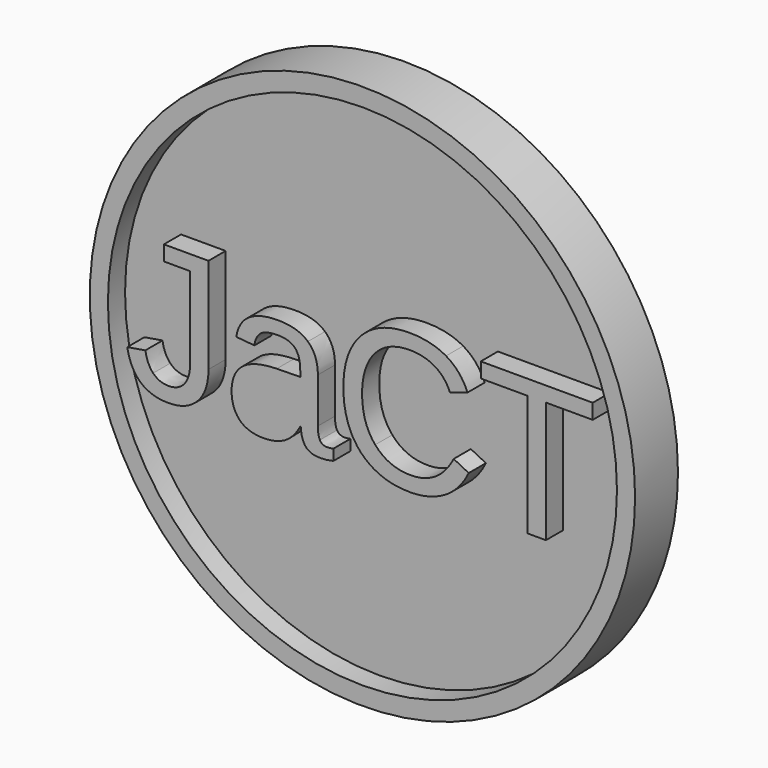
from build123d import *

# Parameters (mm, degrees)
F0_R      = 25.4414928825
F1_DEPTH  = 5
F2_R      = 23.75
F3_DEPTH  = 2
F4_W      = 4.6242554672
F4_H      = 13.1795220077
F5_DEPTH  = 5
F6_R      = 1
F8_D      = 3
F9_W      = 33.4208746554
F9_H      = 3.9936437383
F10_DEPTH = 5
F11_R     = 1.5
F12_R     = 1


with BuildPart() as f1:
    # F0 (on Front) → F1 (new body)
    with BuildSketch(Plane.XZ):
        Circle(F0_R)
    extrude(amount=F1_DEPTH)

    # F2 (on face) → F3 (cut)
    with BuildSketch(Plane.XZ.offset(5)):
        Circle(F2_R)
        with BuildLine():
            add(Edge.make_bspline(
                [(-7.2510674036, -5.9716344181), (-8.0767025075, -6.4364150185), (-9.2574184429, -6.4364150185)],
                knots=[0, 0, 0, 1, 1, 1], degree=2))
            add(Edge.make_bspline(
                [(-9.2574184429, -6.4364150185), (-10.729704817, -6.4364150185), (-11.4687348401, -5.6598561271)],
                knots=[0, 0, 0, 1, 1, 1], degree=2))
            add(Edge.make_bspline(
                [(-11.4687348401, -5.6598561271), (-12.2077648632, -4.8832972356), (-12.2077648632, -3.5293711386)],
                knots=[0, 0, 0, 1, 1, 1], degree=2))
            add(Edge.make_bspline(
                [(-12.2077648632, -3.5293711386), (-12.2077648632, -2.0137822241), (-11.2103630156, -1.2025813003)],
                knots=[0, 0, 0, 1, 1, 1], degree=2))
            add(Edge.make_bspline(
                [(-11.2103630156, -1.2025813003), (-10.212961168, -0.3913803765), (-7.9958710988, -0.336530492)],
                knots=[0, 0, 0, 1, 1, 1], degree=2))
            Line((-7.9958710988, -0.336530492), (-5.8018757177, -0.2990016236))
            Line((-5.8018757177, -0.2990016236), (-5.8018757177, 0.2321762055))
            add(Edge.make_bspline(
                [(-5.8018757177, 0.2321762055), (-5.8018757177, 1.4215526489), (-6.3070720225, 1.9368528798)],
                knots=[0, 0, 0, 1, 1, 1], degree=2))
            add(Edge.make_bspline(
                [(-6.3070720225, 1.9368528798), (-6.8122683274, 2.4521531108), (-7.8948318378, 2.4521531108)],
                knots=[0, 0, 0, 1, 1, 1], degree=2))
            add(Edge.make_bspline(
                [(-7.8948318378, 2.4521531108), (-8.9860558563, 2.4521531108), (-9.482591653, 2.0811946812)],
                knots=[0, 0, 0, 1, 1, 1], degree=2))
            add(Edge.make_bspline(
                [(-9.482591653, 2.0811946812), (-9.9791274498, 1.7102362517), (-10.0801667108, 0.8990353279)],
                knots=[0, 0, 0, 1, 1, 1], degree=2))
            Line((-10.0801667108, 0.8990353279), (-11.774739459, 1.0520376373))
            add(Edge.make_bspline(
                [(-11.774739459, 1.0520376373), (-11.359035071, 3.6877189307), (-7.8601898055, 3.6877189307)],
                knots=[0, 0, 0, 1, 1, 1], degree=2))
            add(Edge.make_bspline(
                [(-7.8601898055, 3.6877189307), (-6.0183884198, 3.6877189307), (-5.0902706369, 2.8433193925)],
                knots=[0, 0, 0, 1, 1, 1], degree=2))
            add(Edge.make_bspline(
                [(-5.0902706369, 2.8433193925), (-4.162152854, 1.9989198544), (-4.162152854, 0.4024995311)],
                knots=[0, 0, 0, 1, 1, 1], degree=2))
            Line((-4.162152854, 0.4024995311), (-4.162152854, -3.8007337252))
            add(Edge.make_bspline(
                [(-4.162152854, -3.8007337252), (-4.162152854, -4.5224427322), (-3.9716216761, -4.8876274897)],
                knots=[0, 0, 0, 1, 1, 1], degree=2))
            add(Edge.make_bspline(
                [(-3.9716216761, -4.8876274897), (-3.7810904983, -5.2528122472), (-3.2499126692, -5.2528122472)],
                knots=[0, 0, 0, 1, 1, 1], degree=2))
            add(Edge.make_bspline(
                [(-3.2499126692, -5.2528122472), (-3.016078951, -5.2528122472), (-2.7187348401, -5.1893018546)],
                knots=[0, 0, 0, 1, 1, 1], degree=2))
            Line((-2.7187348401, -5.1893018546), (-2.7187348401, -6.1996944643))
            add(Edge.make_bspline(
                [(-2.7187348401, -6.1996944643), (-3.330744078, -6.3440362657), (-3.9716216761, -6.3440362657)],
                knots=[0, 0, 0, 1, 1, 1], degree=2))
            add(Edge.make_bspline(
                [(-3.9716216761, -6.3440362657), (-4.8723145168, -6.3440362657), (-5.2836886507, -5.8705951571)],
                knots=[0, 0, 0, 1, 1, 1], degree=2))
            add(Edge.make_bspline(
                [(-5.2836886507, -5.8705951571), (-5.6950627847, -5.3971540486), (-5.7499126692, -4.3867614389)],
                knots=[0, 0, 0, 1, 1, 1], degree=2))
            Line((-5.7499126692, -4.3867614389), (-5.8018757177, -4.3867614389))
            add(Edge.make_bspline(
                [(-5.8018757177, -4.3867614389), (-6.4254322997, -5.5068538176), (-7.2510674036, -5.9716344181)],
                knots=[0, 0, 0, 1, 1, 1], degree=2))
        make_face(mode=Mode.SUBTRACT)
        with BuildLine():
            add(Edge.make_bspline(
                [(-15.3659634775, -5.3755027784), (-16.3676955791, -6.4364150185), (-18.1084577038, -6.4364150185)],
                knots=[0, 0, 0, 1, 1, 1], degree=2))
            add(Edge.make_bspline(
                [(-18.1084577038, -6.4364150185), (-21.3388272188, -6.4364150185), (-21.9421759486, -3.0963457345)],
                knots=[0, 0, 0, 1, 1, 1], degree=2))
            Line((-21.9421759486, -3.0963457345), (-20.2562637085, -2.8163226398))
            add(Edge.make_bspline(
                [(-20.2562637085, -2.8163226398), (-20.0917140549, -3.8642441178), (-19.5244507754, -4.4502718315)],
                knots=[0, 0, 0, 1, 1, 1], degree=2))
            add(Edge.make_bspline(
                [(-19.5244507754, -4.4502718315), (-18.957187496, -5.0362995451), (-18.0997971958, -5.0362995451)],
                knots=[0, 0, 0, 1, 1, 1], degree=2))
            add(Edge.make_bspline(
                [(-18.0997971958, -5.0362995451), (-17.1615754867, -5.0362995451), (-16.6202937316, -4.3910916929)],
                knots=[0, 0, 0, 1, 1, 1], degree=2))
            add(Edge.make_bspline(
                [(-16.6202937316, -4.3910916929), (-16.0790119764, -3.7458838407), (-16.0790119764, -2.5016575128)],
                knots=[0, 0, 0, 1, 1, 1], degree=2))
            Line((-16.0790119764, -2.5016575128), (-16.0790119764, 5.0503055357))
            Line((-16.0790119764, 5.0503055357), (-18.5241620918, 5.0503055357))
            Line((-18.5241620918, 5.0503055357), (-18.5241620918, 6.4561946812))
            Line((-18.5241620918, 6.4561946812), (-14.3642313759, 6.4561946812))
            Line((-14.3642313759, 6.4561946812), (-14.3642313759, -2.4641286444))
            add(Edge.make_bspline(
                [(-14.3642313759, -2.4641286444), (-14.3642313759, -4.3145905382), (-15.3659634775, -5.3755027784)],
                knots=[0, 0, 0, 1, 1, 1], degree=2))
        make_face(mode=Mode.SUBTRACT)
        with BuildLine():
            add(Edge.make_bspline(
                [(6.7500873308, 4.6519221639), (5.7714499174, 5.2379498775), (4.4261843285, 5.2379498775)],
                knots=[0, 0, 0, 1, 1, 1], degree=2))
            add(Edge.make_bspline(
                [(4.4261843285, 5.2379498775), (2.3159071922, 5.2379498775), (1.142408347, 3.8811369445)],
                knots=[0, 0, 0, 1, 1, 1], degree=2))
            add(Edge.make_bspline(
                [(1.142408347, 3.8811369445), (-0.0310904983, 2.5243240115), (-0.0310904983, 0.1600053048)],
                knots=[0, 0, 0, 1, 1, 1], degree=2))
            add(Edge.make_bspline(
                [(-0.0310904983, 0.1600053048), (-0.0310904983, -2.1754450416), (1.1914845594, -3.5972117853)],
                knots=[0, 0, 0, 1, 1, 1], degree=2))
            add(Edge.make_bspline(
                [(1.1914845594, -3.5972117853), (2.4140596172, -5.0189785289), (4.4983552292, -5.0189785289)],
                knots=[0, 0, 0, 1, 1, 1], degree=2))
            add(Edge.make_bspline(
                [(4.4983552292, -5.0189785289), (7.1686785548, -5.0189785289), (8.5139441437, -2.3746367275)],
                knots=[0, 0, 0, 1, 1, 1], degree=2))
            Line((8.5139441437, -2.3746367275), (9.9198332892, -3.0790247183))
            add(Edge.make_bspline(
                [(9.9198332892, -3.0790247183), (9.1346138897, -4.7216344181), (7.7142905641, -5.5790247183)],
                knots=[0, 0, 0, 1, 1, 1], degree=2))
            add(Edge.make_bspline(
                [(7.7142905641, -5.5790247183), (6.2939672384, -6.4364150185), (4.4175238204, -6.4364150185)],
                knots=[0, 0, 0, 1, 1, 1], degree=2))
            add(Edge.make_bspline(
                [(4.4175238204, -6.4364150185), (2.494891026, -6.4364150185), (1.0918887165, -5.6367614389)],
                knots=[0, 0, 0, 1, 1, 1], degree=2))
            add(Edge.make_bspline(
                [(1.0918887165, -5.6367614389), (-0.311113593, -4.8371078592), (-1.045813362, -3.3532741409)],
                knots=[0, 0, 0, 1, 1, 1], degree=2))
            add(Edge.make_bspline(
                [(-1.045813362, -3.3532741409), (-1.7805131311, -1.8694404227), (-1.7805131311, 0.1600053048)],
                knots=[0, 0, 0, 1, 1, 1], degree=2))
            add(Edge.make_bspline(
                [(-1.7805131311, 0.1600053048), (-1.7805131311, 3.199843642), (-0.1379034313, 4.9232847505)],
                knots=[0, 0, 0, 1, 1, 1], degree=2))
            add(Edge.make_bspline(
                [(-0.1379034313, 4.9232847505), (1.5047062684, 6.6467258591), (4.4088633123, 6.6467258591)],
                knots=[0, 0, 0, 1, 1, 1], degree=2))
            add(Edge.make_bspline(
                [(4.4088633123, 6.6467258591), (6.4383090398, 6.6467258591), (7.8008956449, 5.8528459514)],
                knots=[0, 0, 0, 1, 1, 1], degree=2))
            add(Edge.make_bspline(
                [(7.8008956449, 5.8528459514), (9.16348225, 5.0589660438), (9.8043598481, 3.4971877528)],
                knots=[0, 0, 0, 1, 1, 1], degree=2))
            Line((9.8043598481, 3.4971877528), (8.1704106564, 2.9573494156))
            add(Edge.make_bspline(
                [(8.1704106564, 2.9573494156), (7.7287247442, 4.0658944503), (6.7500873308, 4.6519221639)],
                knots=[0, 0, 0, 1, 1, 1], degree=2))
        make_face(mode=Mode.SUBTRACT)
        Polygon((21.4873852523, 5.0503055357), (17.1196023424, 5.0503055357), (17.1196023424, -6.2545443488), (15.4048217419, -6.2545443488), (15.4048217419, 5.0503055357), (11.039925668, 5.0503055357), (11.039925668, 6.4561946812), (21.4873852523, 6.4561946812), align=None, mode=Mode.SUBTRACT)
    extrude(amount=-F3_DEPTH, mode=Mode.SUBTRACT)

    # F4 (on face) → F5 (join)
    with BuildSketch(Plane(origin=(0, 0, 0), x_dir=(-1, 0, 0), z_dir=(0, 1, 0))):
        with Locations((8.8527675252, 6.5897610039)):
            Rectangle(F4_W, F4_H)
    extrude(amount=F5_DEPTH)

    # F6
    f6_edges = [f1.edges().sort_by_distance(p)[0] for p in [
        (-8.852768, 5, 13.179522),
        (-6.54064, 5, 6.589761),
        (-8.852768, 5, 0),
        (-11.164895, 5, 6.589761),
    ]]
    fillet(f6_edges, radius=F6_R)

    # F8 (through all)
    with Locations(Plane(origin=(0, 0, 0), x_dir=(1, 0, 0), z_dir=(0, 0, -1))):
        with Locations((-8.9718680829, -1.9239948597)):
            Hole(F8_D / 2)

    # F9 (on face) → F10 (join)
    with BuildSketch(Plane(origin=(0, 0, 0), x_dir=(-1, 0, 0), z_dir=(0, 1, 0))):
        with Locations((0, -17.1873081453)):
            Rectangle(F9_W, F9_H)
    extrude(amount=F10_DEPTH)

    # F11
    f11_edges = [f1.edges().sort_by_distance(p)[0] for p in [
        (0, 5, -15.190486),
        (0, 5, -19.18413),
    ]]
    fillet(f11_edges, radius=F11_R)

    # F12
    f12_edges = [f1.edges().sort_by_distance(p)[0] for p in [
        (16.710437, 5, -17.187308),
        (-16.710437, 5, -17.187308),
    ]]
    fillet(f12_edges, radius=F12_R)


solid = f1.part
